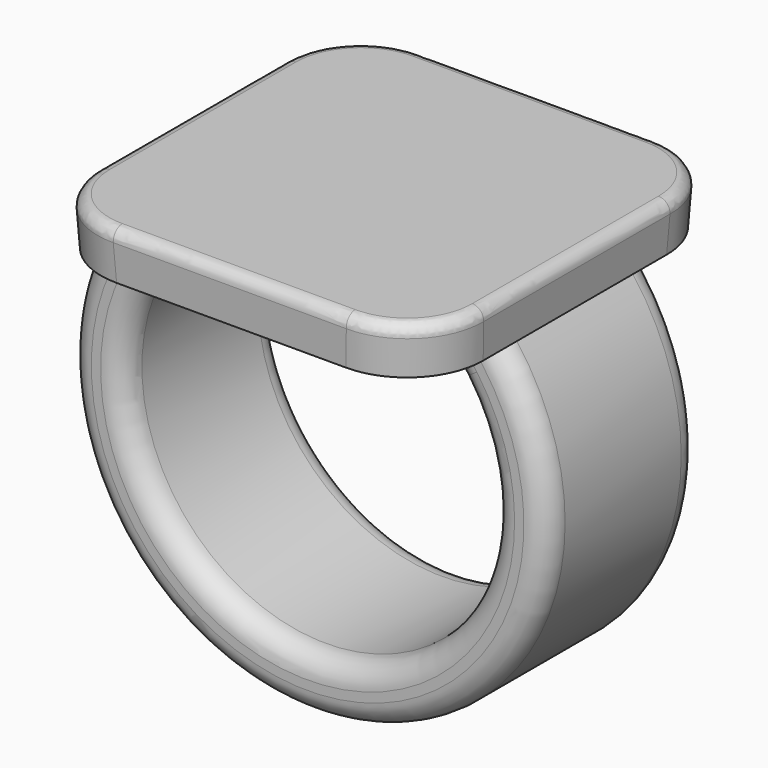
from build123d import *

# Parameters (mm, degrees)
F0_W          = 25.4
F0_H          = 25.4
F1_DEPTH      = 3.175
F1_TAPER      = -3
F3_W          = 5.08
F3_H          = 12.7
F6_DEPTH      = 6.35
F6_DEPTH_BACK = 6.35
F7_R          = 5.08
F8_R          = 1.524
F9_R          = 0.762


with BuildPart() as f1:
    # F0 (on Top) → F1 (new body)
    with BuildSketch(Plane.XY):
        Rectangle(F0_W, F0_H)
    extrude(amount=F1_DEPTH, taper=F1_TAPER)

    # F4: sweep along a path in F2
    with BuildLine(Plane.XZ) as f4_path:
        ThreePointArc((-10.16, 0), (0, -23.5582897328), (10.16, 0))
    # F3 (on face) → F4 (sweep)
    with BuildSketch(Plane(origin=(0, 0, 0), x_dir=(1, 0, 0), z_dir=(0, 0, -1))):
        with Locations((-10.16, 0)):
            Rectangle(F3_W, F3_H)
    sweep(path=f4_path.line)

    # F5 (on Front) → F6 (join, two sides)
    with BuildSketch(Plane.XZ) as f6_sk:
        with BuildLine():
            Line((10.0130578512, -2.535746045), (10.16, 0))
            Line((10.16, 0), (7.62, 0))
            ThreePointArc((7.62, 0), (8.9072265211, -1.1822790439), (10.0130578512, -2.535746045))
        make_face()
    extrude(amount=F6_DEPTH)
    extrude(f6_sk.sketch, amount=-F6_DEPTH_BACK)

    # F7
    f7_edges = [f1.edges().sort_by_distance(p)[0] for p in [
        (12.783197, -12.783197, 1.5875),
        (12.783197, 12.783197, 1.5875),
        (-12.783197, 12.783197, 1.5875),
        (-12.783197, -12.783197, 1.5875),
    ]]
    fillet(f7_edges, radius=F7_R)

    # F8
    f8_edges = [f1.edges().sort_by_distance(p)[0] for p in [
        (-1.743325, -6.35, -21.711017),
        (8.907227, -6.35, -1.182279),
        (-1.743325, 6.35, -21.711017),
        (0, 6.35, -25.501344),
        (0, -6.35, -25.501344),
        (8.907227, 6.35, -1.182279),
    ]]
    fillet(f8_edges, radius=F8_R)

    # F9
    f9_edges = [f1.edges().sort_by_distance(p)[0] for p in [
        (0, -12.866395, 3.175),
        (-11.381378, -11.381378, 3.175),
        (12.866395, 0, 3.175),
        (11.381378, -11.381378, 3.175),
        (11.381378, 11.381378, 3.175),
        (0, 12.866395, 3.175),
        (-11.381378, 11.381378, 3.175),
        (-12.866395, 0, 3.175),
    ]]
    fillet(f9_edges, radius=F9_R)


solid = f1.part
